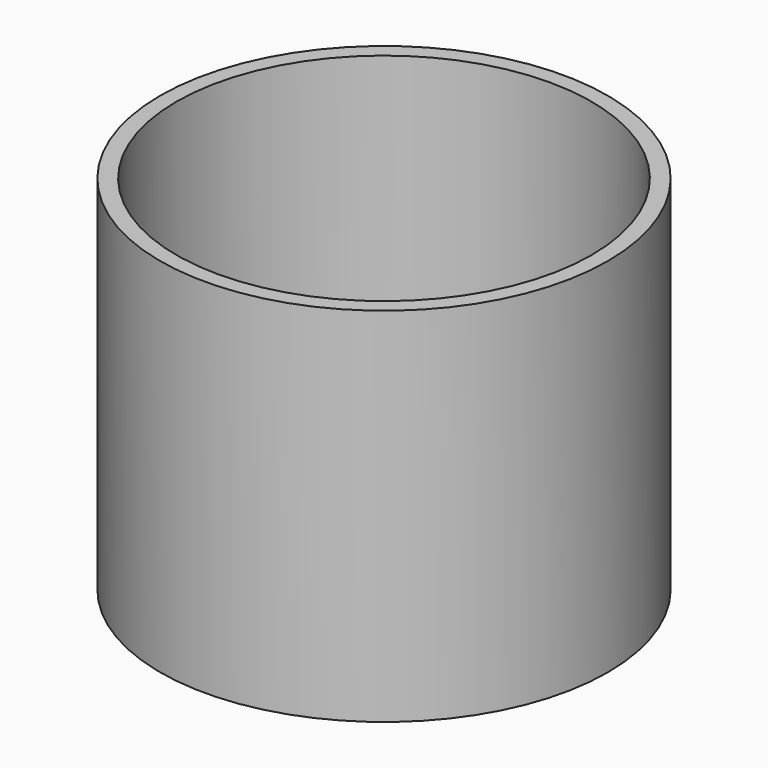
from build123d import *

# Parameters (mm, degrees)
F0_R     = 30
F0_R_2   = 25
F1_DEPTH = 200
F3_R     = 340.0421742973
F3_R_2   = 315.4048789829
F4_DEPTH = 550
F2_R     = 25
F2_R_2   = 24
F5_DEPTH = 5
F6_R     = 25
F6_R_2   = 24
F7_DEPTH = 5
F8_R     = 24
F8_R_2   = 23
F9_DEPTH = 160


with BuildPart() as f1:
    # F0 (on Top) → F1 (new body)
    with BuildSketch(Plane.XY):
        Circle(F0_R)
        Circle(F0_R_2, mode=Mode.SUBTRACT)
    extrude(amount=F1_DEPTH)

    # F2 (on face) → F5 (join)
    with BuildSketch(Plane.XY.offset(200)):
        Circle(F2_R)
        Circle(F2_R_2, mode=Mode.SUBTRACT)
    extrude(amount=-F5_DEPTH)


with BuildPart() as f4:
    # F3 (on Top) → F4 (new body)
    with BuildSketch(Plane.XY):
        Circle(F3_R)
        Circle(F3_R_2, mode=Mode.SUBTRACT)
    extrude(amount=F4_DEPTH)


with BuildPart() as f7:
    # F6 (on face) → F7 (new body)
    with BuildSketch(Plane(origin=(0, 0, 195), x_dir=(1, 0, 0), z_dir=(0, 0, -1))):
        Circle(F6_R)
        Circle(F6_R_2, mode=Mode.SUBTRACT)
    extrude(amount=F7_DEPTH)

    # F8 (on face) → F9 (join)
    with BuildSketch(Plane(origin=(0, 0, 190), x_dir=(1, 0, 0), z_dir=(0, 0, -1))):
        Circle(F8_R)
        Circle(F8_R_2, mode=Mode.SUBTRACT)
    extrude(amount=-F9_DEPTH)


solid = Compound([f1.part, f4.part, f7.part])
